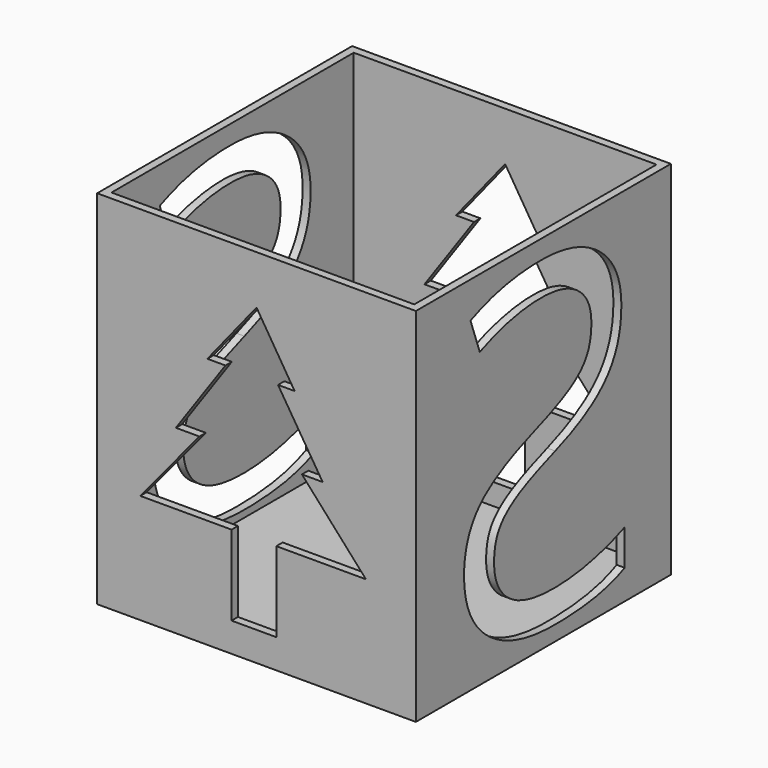
from build123d import *

# Parameters (mm, degrees)
F0_W         = 100
F0_H         = 113.5
F1_DEPTH     = 50
F2_T         = -2.5
F3_W         = 14.021969866
F3_H         = 25.1343827695
F4_DEPTH     = 100.001
F5_TEXT_SIZE = 140.2344037261
F6_DEPTH     = 100.001


# Not quite as in the source:
# - Text() gives the source's letters only with a copy of the font that has no kerning and outlines rounded to 1/6400 em; it was checked with that copy


with BuildPart() as f1:
    # F0 (on Front) → F1 (new body, symmetric)
    with BuildSketch(Plane.XZ):
        Rectangle(F0_W, F0_H)
    extrude(amount=F1_DEPTH, both=True)

    # F2
    f2_openings = [f1.faces().sort_by_distance(p)[0] for p in [
        (0, 0, 56.75),
    ]]
    offset(amount=F2_T, openings=f2_openings)

    # F3 (on face) → F4 (cut, through all)
    with BuildSketch(Plane.XZ.offset(50)):
        Polygon((-9.7508355975, 22.2730264068), (6.7500988953, 22.2730264068), (11.9573445991, 22.2730264068), (0, 41.4573661983), (-15.4131352901, 22.2730264068), align=None)
        Polygon((-17.9065223783, 0), (14.2429284751, 0), (20.7514669746, 0), (6.7500988953, 22.2730264068), (-9.7508355975, 22.2730264068), (-25.3045689315, 0), align=None)
        Polygon((-7.8152241185, -22.4434416741), (6.2067457475, -22.4434416741), (34.3286842108, -22.4434416741), (14.2429284751, 0), (-17.9065223783, 0), (-36.4849381149, -22.4434416741), align=None)
        with Locations((-0.8042391855, -35.0106330588)):
            Rectangle(F3_W, F3_H)
    extrude(amount=-F4_DEPTH, mode=Mode.SUBTRACT)

    # F5 (on face) → F6 (cut, through all)
    with BuildSketch(Plane(origin=(-50, 0, 0), x_dir=(0, -1, 0), z_dir=(-1, 0, 0))):
        with Locations((-39.1511507332, -50.6904453796)):
            Text('S', F5_TEXT_SIZE, font='Open Sans', text_align=(TextAlign.LEFT, TextAlign.BOTTOM))
    extrude(amount=-F6_DEPTH, mode=Mode.SUBTRACT)


solid = f1.part
